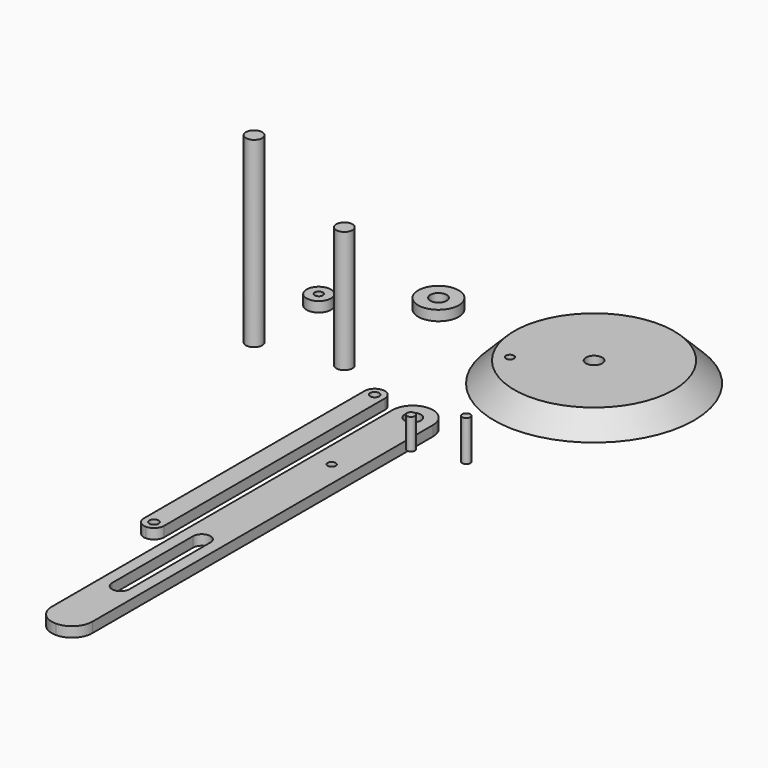
from build123d import *

# Parameters (mm, degrees)
F0_R      = 49.315
F1_DEPTH  = 10
F2_SIZE   = 9.99999
F3_R      = 4
F3_R_2    = 2
F4_DEPTH  = 10.001
F5_R      = 10
F6_DEPTH  = 5
F5_R_2    = 6
F7_R      = 4
F8_DEPTH  = 5.001
F9_R      = 4
F10_DEPTH = 60
F11_R     = 2
F12_DEPTH = 5.001
F13_W     = 10
F13_H     = 5
F14_DEPTH = 146
F15_R     = 4.99999
F16_R     = 2.25
F17_DEPTH = 5.001
F18_W     = 20
F18_H     = 5
F19_DEPTH = 230
F20_R     = 9.99999
F21_R     = 4
F22_DEPTH = 5.001
F23_R     = 2
F24_DEPTH = 5.001
F25_R     = 4
F26_DEPTH = 90
F27_R     = 2
F28_DEPTH = 15
F29_R     = 2
F30_DEPTH = 20


# Not quite as in the source:
# - a fillet or chamfer is up to 0.001 mm smaller than in the source, because OpenCascade refuses the exact size


with BuildPart() as f1:
    # F0 (on Top) → F1 (new body)
    with BuildSketch(Plane.XY):
        with Locations((35.7543155551, 29.4181052595)):
            Circle(F0_R)
    extrude(amount=F1_DEPTH)

    # F2 (size 10 in the source; OpenCascade refuses exactly that, so slightly less here)
    f2_edges = [f1.edges().sort_by_distance(p)[0] for p in [
        (-13.560684, 29.418105, 10),
    ]]
    chamfer(f2_edges, length=F2_SIZE)

    # F3 (on face) → F4 (cut, through all)
    with BuildSketch(Plane.XY.offset(10)):
        with Locations((35.7543155551, 29.4181052595)):
            Circle(F3_R)
        with Locations((8.7423292544, 11.3459555233)):
            Circle(F3_R_2)
    extrude(amount=-F4_DEPTH, mode=Mode.SUBTRACT)


with BuildPart() as f6:
    # F5 (on Top) → F6 (new body)
    with BuildSketch(Plane.XY):
        with Locations((-49.6336221695, 40.280174464)):
            Circle(F5_R)
    extrude(amount=F6_DEPTH)

    # F7 (on face) → F8 (cut, through all)
    with BuildSketch(Plane.XY.offset(5)):
        with Locations((-49.6336221695, 40.280174464)):
            Circle(F7_R)
    extrude(amount=-F8_DEPTH, mode=Mode.SUBTRACT)


with BuildPart() as f6b:
    # F5 (on Top) → F6, piece 2 (new body)
    with BuildSketch(Plane.XY):
        with Locations((-87.6508653164, 14.0301734209)):
            Circle(F5_R_2)
    extrude(amount=F6_DEPTH)

    # F11 (on face) → F12 (cut, through all)
    with BuildSketch(Plane.XY.offset(5)):
        with Locations((-87.6508653164, 14.0301734209)):
            Circle(F11_R)
    extrude(amount=-F12_DEPTH, mode=Mode.SUBTRACT)


with BuildPart() as f10:
    # F9 (on Top) → F10 (new body)
    with BuildSketch(Plane.XY):
        with Locations((-48.7284511328, -18.8577584922)):
            Circle(F9_R)
    extrude(amount=F10_DEPTH)


with BuildPart() as f14:
    # F13 (on Front) → F14 (new body)
    with BuildSketch(Plane.XZ):
        with Locations((-44.8726732284, -19.596266548)):
            Rectangle(F13_W, F13_H)
    extrude(amount=F14_DEPTH)

    # F15 (radius 5 in the source; OpenCascade refuses exactly that, so slightly less here)
    f15_edges = [f14.edges().sort_by_distance(p)[0] for p in [
        (-49.872673, -146, -19.596267),
        (-39.872673, -146, -19.596267),
        (-39.872673, 0, -19.596267),
        (-49.872673, 0, -19.596267),
    ]]
    fillet(f15_edges, radius=F15_R)

    # F16 (on face) → F17 (cut, through all)
    with BuildSketch(Plane.XY.offset(-17.096266548)):
        with Locations((-44.8726732284, -5)):
            Circle(F16_R)
        with Locations((-44.8726732284, -141)):
            Circle(F16_R)
    extrude(amount=-F17_DEPTH, mode=Mode.SUBTRACT)


with BuildPart() as f19:
    # F18 (on Front) → F19 (new body)
    with BuildSketch(Plane.XZ):
        with Locations((-22.0925002359, -20.0699501518)):
            Rectangle(F18_W, F18_H)
    extrude(amount=F19_DEPTH)

    # F20 (radius 10 in the source; OpenCascade refuses exactly that, so slightly less here)
    f20_edges = [f19.edges().sort_by_distance(p)[0] for p in [
        (-32.0925, -230, -20.06995),
        (-12.0925, -230, -20.06995),
        (-32.0925, 0, -20.06995),
        (-12.0925, 0, -20.06995),
    ]]
    fillet(f20_edges, radius=F20_R)

    # F21 (on face) → F22 (cut, through all)
    with BuildSketch(Plane.XY.offset(-17.5699501518)):
        with Locations((-22.0925002359, -10)):
            Circle(F21_R)
        with BuildLine():
            ThreePointArc((-26.3425002359, -140), (-22.0925002359, -144.25), (-17.8425002359, -140))
            ThreePointArc((-17.8425002359, -140), (-22.0925002359, -135.75), (-26.3425002359, -140))
        make_face()
        with BuildLine():
            Line((-17.8425002359, -190), (-17.8425002359, -140))
            ThreePointArc((-17.8425002359, -140), (-22.0925002359, -144.25), (-26.3425002359, -140))
            Line((-26.3425002359, -140), (-26.3425002359, -190))
            ThreePointArc((-26.3425002359, -190), (-22.0925002359, -185.75), (-17.8425002359, -190))
        make_face()
        with BuildLine():
            ThreePointArc((-26.3425002359, -190), (-22.0925002359, -194.25), (-17.8425002359, -190))
            ThreePointArc((-17.8425002359, -190), (-22.0925002359, -185.75), (-26.3425002359, -190))
        make_face()
    extrude(amount=-F22_DEPTH, mode=Mode.SUBTRACT)

    # F23 (on face) → F24 (cut, through all)
    with BuildSketch(Plane.XY.offset(-17.5699501518)):
        with Locations((-22.0925002359, -60)):
            Circle(F23_R)
    extrude(amount=-F24_DEPTH, mode=Mode.SUBTRACT)


with BuildPart() as f26:
    # F25 (on Top) → F26 (new body)
    with BuildSketch(Plane.XY):
        with Locations((-87.817274034, -25.6417505443)):
            Circle(F25_R)
    extrude(amount=F26_DEPTH)


with BuildPart() as f28:
    # F27 (on Top) → F28 (new body)
    with BuildSketch(Plane.XY):
        with Locations((14.9050457403, -57.3387555778)):
            Circle(F27_R)
    extrude(amount=F28_DEPTH)


with BuildPart() as f30:
    # F29 (on Top) → F30 (new body)
    with BuildSketch(Plane.XY):
        with Locations((38.122959435, -52.2697754204)):
            Circle(F29_R)
    extrude(amount=F30_DEPTH)


solid = Compound([f1.part, f6.part, f6b.part, f10.part, f14.part, f19.part, f26.part, f28.part, f30.part])
